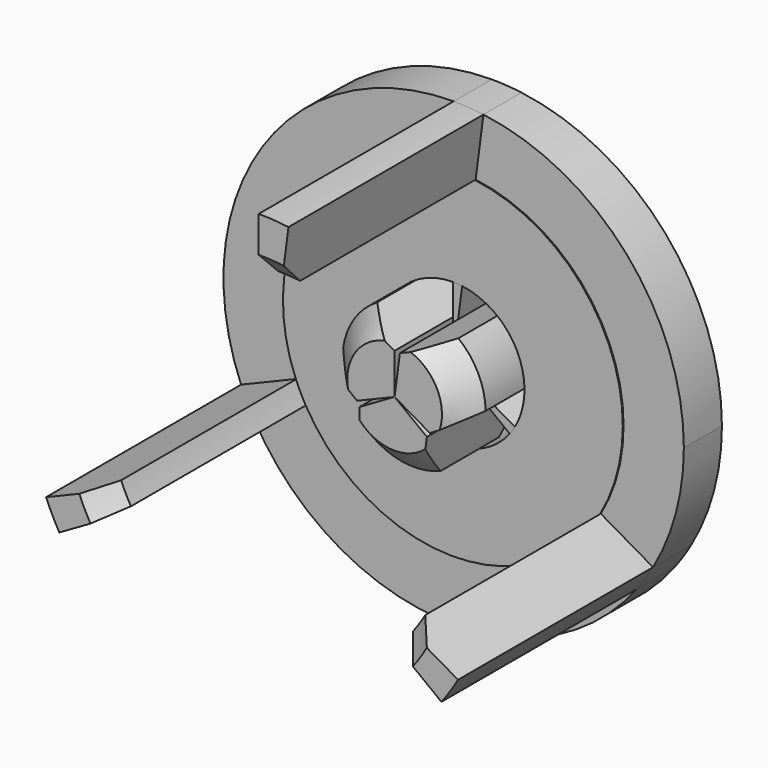
from build123d import *

# Parameters (mm, degrees)
F1_DEPTH      = 60
F2_DEPTH      = 9.8
F3_DEPTH      = 25
F4_DEPTH      = 10
F5_DEPTH      = 10
F6_T1_DEPTH   = 64.9472775058
F6_T4_ANGLE   = 212.5191011757
F6_T6_ANGLE   = 212.5191011757
F6_2_T1_DEPTH = 64.9472775058
F6_2_T4_ANGLE = 212.5191011757
F6_2_T6_ANGLE = 212.5191011757
F6_3_T1_DEPTH = 64.9472775058
F6_3_T4_ANGLE = 212.5191011757
F6_3_T6_ANGLE = 212.5191011757
F7_SIZE       = 5
F7_2_SIZE     = 5
F7_3_SIZE     = 5


# Not quite as in the source:
# - a fillet or chamfer that OpenCascade refuses, or shapes differently, is made with other operations: its cross-section is extruded or revolved along the edge and cut away or added


with BuildPart() as f1:
    # F0 (on Front) → F1 (new body)
    with BuildSketch(Plane.XZ):
        with BuildLine():
            ThreePointArc((0, 35), (2.2707204157, 34.9262627373), (4.5318730195, 34.7053616454))
            Line((4.5318730195, 34.7053616454), (6.1392555161, 47.0147954288))
            ThreePointArc((6.1392555161, 47.0147954288), (3.0761084385, 47.3140465864), (0, 47.4139372706))
            Line((0, 47.4139372706), (0, 35))
        make_face()
    extrude(amount=F1_DEPTH)

    # F7
    f7_edges = [f1.edges().sort_by_distance(p)[0] for p in [
        (2.27072, -60, 34.926263),
    ]]
    chamfer(f7_edges, length=F7_SIZE)


with BuildPart() as f1b:
    # F0 (on Front) → F1, piece 2 (new body)
    with BuildSketch(Plane.XZ):
        with BuildLine():
            Line((41.0616741698, -23.7069686353), (30.3108891325, -17.5))
            ThreePointArc((30.3108891325, -17.5), (29.1116705819, -19.4296329335), (27.7897883227, -21.2773979843))
            Line((27.7897883227, -21.2773979843), (37.646379437, -28.8241489517))
            ThreePointArc((37.646379437, -28.8241489517), (39.4371120804, -26.3210113457), (41.0616741698, -23.7069686353))
        make_face()
    extrude(amount=F1_DEPTH)

    # F7#2
    f7_2_edges = [f1b.edges().sort_by_distance(p)[0] for p in [
        (29.111671, -60, -19.429633),
    ]]
    chamfer(f7_2_edges, length=F7_2_SIZE)


with BuildPart() as f1c:
    # F0 (on Front) → F1, piece 3 (new body)
    with BuildSketch(Plane.XZ):
        with BuildLine():
            ThreePointArc((-30.3108891325, -17.5), (-31.3823909976, -15.4966298038), (-32.3216613422, -13.4279636611))
            Line((-32.3216613422, -13.4279636611), (-43.7856349531, -18.1906464771))
            ThreePointArc((-43.7856349531, -18.1906464771), (-42.5132205189, -20.9930352406), (-41.0616741698, -23.7069686353))
            Line((-41.0616741698, -23.7069686353), (-30.3108891325, -17.5))
        make_face()
    extrude(amount=F1_DEPTH)

    # F7#3
    f7_3_edges = [f1c.edges().sort_by_distance(p)[0] for p in [
        (-31.382391, -60, -15.49663),
    ]]
    chamfer(f7_3_edges, length=F7_3_SIZE)


with BuildPart() as f2:
    # F0 (on Front) → F2 (new body)
    with BuildSketch(Plane.XZ):
        with BuildLine():
            ThreePointArc((4.5318730195, 34.7053616454), (26.3022390271, 23.0909554189), (35, 0))
            ThreePointArc((35, 0), (33.8074039201, -9.0586665786), (30.3108891325, -17.5))
            Line((30.3108891325, -17.5), (41.0616741698, -23.7069686353))
            ThreePointArc((41.0616741698, -23.7069686353), (45.7983465358, -12.2716299689), (47.4139372706, 0))
            ThreePointArc((47.4139372706, 0), (35.6312203232, 31.2809460501), (6.1392555161, 47.0147954288))
            Line((6.1392555161, 47.0147954288), (4.5318730195, 34.7053616454))
        make_face()
        with BuildLine():
            ThreePointArc((0, 35), (2.2707204157, 34.9262627373), (4.5318730195, 34.7053616454))
            Line((4.5318730195, 34.7053616454), (6.1392555161, 47.0147954288))
            ThreePointArc((6.1392555161, 47.0147954288), (3.0761084385, 47.3140465864), (0, 47.4139372706))
            Line((0, 47.4139372706), (0, 35))
        make_face()
        with BuildLine():
            Line((41.0616741698, -23.7069686353), (30.3108891325, -17.5))
            ThreePointArc((30.3108891325, -17.5), (29.1116705819, -19.4296329335), (27.7897883227, -21.2773979843))
            Line((27.7897883227, -21.2773979843), (37.646379437, -28.8241489517))
            ThreePointArc((37.646379437, -28.8241489517), (39.4371120804, -26.3210113457), (41.0616741698, -23.7069686353))
        make_face()
        with BuildLine():
            ThreePointArc((-32.3216613422, -13.4279636611), (-29.1116705819, 19.4296329335), (0, 35))
            Line((0, 35), (0, 47.4139372706))
            ThreePointArc((0, 47.4139372706), (-39.4371120804, 26.3210113457), (-43.7856349531, -18.1906464771))
            Line((-43.7856349531, -18.1906464771), (-32.3216613422, -13.4279636611))
        make_face()
        with BuildLine():
            Line((37.646379437, -28.8241489517), (27.7897883227, -21.2773979843))
            ThreePointArc((27.7897883227, -21.2773979843), (-2.2707204157, -34.9262627373), (-30.3108891325, -17.5))
            Line((-30.3108891325, -17.5), (-41.0616741698, -23.7069686353))
            ThreePointArc((-41.0616741698, -23.7069686353), (-3.0761084385, -47.3140465864), (37.646379437, -28.8241489517))
        make_face()
        with BuildLine():
            ThreePointArc((-30.3108891325, -17.5), (-31.3823909976, -15.4966298038), (-32.3216613422, -13.4279636611))
            Line((-32.3216613422, -13.4279636611), (-43.7856349531, -18.1906464771))
            ThreePointArc((-43.7856349531, -18.1906464771), (-42.5132205189, -20.9930352406), (-41.0616741698, -23.7069686353))
            Line((-41.0616741698, -23.7069686353), (-30.3108891325, -17.5))
        make_face()
    extrude(amount=F2_DEPTH)


with BuildPart() as f3:
    # F0 (on Front) → F3 (new body)
    with BuildSketch(Plane.XZ):
        with BuildLine():
            Line((0, 0), (0, 14.75))
            ThreePointArc((0, 14.75), (-12.2684897452, 8.1882024506), (-13.6212715656, -5.6589275429))
            Line((-13.6212715656, -5.6589275429), (0, 0))
        make_face()
    extrude(amount=F3_DEPTH)

    # F6: chamfer of 5 on 4 edges, made by hand

    # F6_s2 → F6_t1 (cut)
    with BuildSketch(Plane.XZ.offset(-19.9736387529)):
        with BuildLine():
            Line((0, 8.3703345214), (-7.5641025641, 12.6628137631))
            ThreePointArc((-7.5641025641, 12.6628137631), (-3.9937030678, 14.1990434821), (0, 14.75))
            Line((0, 14.75), (0, 8.3703345214))
        make_face()
        with BuildLine():
            Line((-7.7298033635, -3.2113299367), (-14.5958192129, 2.1271016679))
            ThreePointArc((-14.5958192129, 2.1271016679), (-14.6446849851, -1.759460624), (-13.6212715656, -5.6589275429))
            Line((-13.6212715656, -5.6589275429), (-7.7298033635, -3.2113299367))
        make_face()
    extrude(amount=F6_T1_DEPTH, mode=Mode.SUBTRACT)

    # F6_s3 → F6_t4 (revolve, cut)
    with BuildSketch(Plane(origin=(0, 0, 0), x_dir=(0, 1, 0), z_dir=(0.6430632155, 0, -0.7658130979))):
        Polygon((-5, 14.75), (0, 9.75), (0, 14.75), align=None)
    revolve(axis=Axis((0, 0, 0), (0, -1, 0)), revolution_arc=F6_T4_ANGLE, mode=Mode.SUBTRACT)

    # F6_s5 → F6_t6 (revolve, cut)
    with BuildSketch(Plane(origin=(0, 0, 0), x_dir=(0, 1, 0), z_dir=(0.6430632155, 0, -0.7658130979))):
        Polygon((-20, 14.75), (-25, 9.75), (-25, 14.75), align=None)
    revolve(axis=Axis((0, -25, 0), (0, -1, 0)), revolution_arc=F6_T6_ANGLE, mode=Mode.SUBTRACT)


with BuildPart() as f3b:
    # F0 (on Front) → F3, piece 2 (new body)
    with BuildSketch(Plane.XZ):
        with BuildLine():
            ThreePointArc((14.75, 0), (11.0845150186, 9.7311883551), (1.9098607725, 14.6258309791))
            Line((1.9098607725, 14.6258309791), (0, 0))
            Line((0, 0), (12.7738747058, -7.375))
            ThreePointArc((12.7738747058, -7.375), (14.2474059378, -3.8175809153), (14.75, 0))
        make_face()
    extrude(amount=F3_DEPTH)

    # F6#2: chamfer of 5 on 4 edges, made by hand

    # F6_2_s2 → F6_2_t1 (cut)
    with BuildSketch(Plane.XZ.offset(-19.9736387529)):
        with BuildLine():
            Line((7.2489223337, -4.1851672607), (14.7483696843, 0.2192980958))
            ThreePointArc((14.7483696843, 0.2192980958), (14.2935838988, -3.6408734291), (12.7738747058, -7.375))
            Line((12.7738747058, -7.375), (7.2489223337, -4.1851672607))
        make_face()
        with BuildLine():
            Line((1.0838083766, 8.2998710474), (9.1400336873, 11.5767993934))
            ThreePointArc((9.1400336873, 11.5767993934), (5.7986048952, 13.5623995395), (1.9098607725, 14.6258309791))
            Line((1.9098607725, 14.6258309791), (1.0838083766, 8.2998710474))
        make_face()
    extrude(amount=F6_2_T1_DEPTH, mode=Mode.SUBTRACT)

    # F6_2_s3 → F6_2_t4 (revolve, cut)
    with BuildSketch(Plane(origin=(0, 0, 0), x_dir=(0, 1, 0), z_dir=(-0.7368088334, 0, -0.6761011337))):
        Polygon((-25, -9.75), (-20, -14.75), (-25, -14.75), align=None)
    revolve(axis=Axis((0, -25, 0), (0, 1, 0)), revolution_arc=F6_2_T4_ANGLE, mode=Mode.SUBTRACT)

    # F6_2_s5 → F6_2_t6 (revolve, cut)
    with BuildSketch(Plane(origin=(0, 0, 0), x_dir=(0, 1, 0), z_dir=(-0.9847452051, 0, -0.1740025319))):
        Polygon((0, 9.75), (-5, 14.75), (0, 14.75), align=None)
    revolve(axis=Axis((0, 0, 0), (0, -1, 0)), revolution_arc=F6_2_T6_ANGLE, mode=Mode.SUBTRACT)


with BuildPart() as f3c:
    # F0 (on Front) → F3, piece 3 (new body)
    with BuildSketch(Plane.XZ):
        with BuildLine():
            Line((11.7114107931, -8.9669034362), (0, 0))
            Line((0, 0), (-12.7738747058, -7.375))
            ThreePointArc((-12.7738747058, -7.375), (-0.9569464609, -14.7189250107), (11.7114107931, -8.9669034362))
        make_face()
    extrude(amount=F3_DEPTH)

    # F6#3: chamfer of 5 on 4 edges, made by hand

    # F6_3_s2 → F6_3_t1 (cut)
    with BuildSketch(Plane.XZ.offset(-19.9736387529)):
        with BuildLine():
            Line((-7.2489223337, -4.1851672607), (-7.1842671202, -12.8821118589))
            ThreePointArc((-7.1842671202, -12.8821118589), (-10.299880831, -10.558170053), (-12.7738747058, -7.375))
            Line((-12.7738747058, -7.375), (-7.2489223337, -4.1851672607))
        make_face()
        with BuildLine():
            Line((6.6459949868, -5.0885411107), (5.4557855256, -13.7039010613))
            ThreePointArc((5.4557855256, -13.7039010613), (8.8460800899, -11.8029389155), (11.7114107931, -8.9669034362))
            Line((11.7114107931, -8.9669034362), (6.6459949868, -5.0885411107))
        make_face()
    extrude(amount=F6_3_T1_DEPTH, mode=Mode.SUBTRACT)

    # F6_3_s3 → F6_3_t4 (revolve, cut)
    with BuildSketch(Plane(origin=(0, 0, 0), x_dir=(0, 1, 0), z_dir=(0.3416819896, 0, 0.9398156298))):
        Polygon((-20, 14.75), (-25, 9.75), (-25, 14.75), align=None)
    revolve(axis=Axis((0, -25, 0), (0, -1, 0)), revolution_arc=F6_3_T4_ANGLE, mode=Mode.SUBTRACT)

    # F6_3_s5 → F6_3_t6 (revolve, cut)
    with BuildSketch(Plane(origin=(0, 0, 0), x_dir=(0, 1, 0), z_dir=(0.3416819896, 0, 0.9398156298))):
        Polygon((-5, 14.75), (0, 9.75), (0, 14.75), align=None)
    revolve(axis=Axis((0, 0, 0), (0, -1, 0)), revolution_arc=F6_3_T6_ANGLE, mode=Mode.SUBTRACT)


with BuildPart() as f4:
    # F0 (on Front) → F4 (new body)
    with BuildSketch(Plane.XZ):
        with BuildLine():
            ThreePointArc((-30.3108891325, -17.5), (-2.2707204157, -34.9262627373), (27.7897883227, -21.2773979843))
            Line((27.7897883227, -21.2773979843), (11.7114107931, -8.9669034362))
            ThreePointArc((11.7114107931, -8.9669034362), (-0.9569464609, -14.7189250107), (-12.7738747058, -7.375))
            Line((-12.7738747058, -7.375), (-30.3108891325, -17.5))
        make_face()
        with BuildLine():
            ThreePointArc((30.3108891325, -17.5), (33.8074039201, -9.0586665786), (35, 0))
            ThreePointArc((35, 0), (26.3022390271, 23.0909554189), (4.5318730195, 34.7053616454))
            Line((4.5318730195, 34.7053616454), (1.9098607725, 14.6258309791))
            ThreePointArc((1.9098607725, 14.6258309791), (11.0845150186, 9.7311883551), (14.75, 0))
            ThreePointArc((14.75, 0), (14.2474059378, -3.8175809153), (12.7738747058, -7.375))
            Line((12.7738747058, -7.375), (30.3108891325, -17.5))
        make_face()
        with BuildLine():
            ThreePointArc((27.7897883227, -21.2773979843), (29.1116705819, -19.4296329335), (30.3108891325, -17.5))
            Line((30.3108891325, -17.5), (12.7738747058, -7.375))
            ThreePointArc((12.7738747058, -7.375), (12.2684897452, -8.1882024506), (11.7114107931, -8.9669034362))
            Line((11.7114107931, -8.9669034362), (27.7897883227, -21.2773979843))
        make_face()
        with BuildLine():
            Line((-13.6212715656, -5.6589275429), (-32.3216613422, -13.4279636611))
            ThreePointArc((-32.3216613422, -13.4279636611), (-31.3823909976, -15.4966298038), (-30.3108891325, -17.5))
            Line((-30.3108891325, -17.5), (-12.7738747058, -7.375))
            ThreePointArc((-12.7738747058, -7.375), (-13.2254362061, -6.5307225602), (-13.6212715656, -5.6589275429))
        make_face()
        with BuildLine():
            Line((0, 14.75), (0, 35))
            ThreePointArc((0, 35), (-29.1116705819, 19.4296329335), (-32.3216613422, -13.4279636611))
            Line((-32.3216613422, -13.4279636611), (-13.6212715656, -5.6589275429))
            ThreePointArc((-13.6212715656, -5.6589275429), (-12.2684897452, 8.1882024506), (0, 14.75))
        make_face()
        with BuildLine():
            Line((1.9098607725, 14.6258309791), (4.5318730195, 34.7053616454))
            ThreePointArc((4.5318730195, 34.7053616454), (2.2707204157, 34.9262627373), (0, 35))
            Line((0, 35), (0, 14.75))
            ThreePointArc((0, 14.75), (0.9569464609, 14.7189250107), (1.9098607725, 14.6258309791))
        make_face()
    extrude(amount=F4_DEPTH)


with BuildPart() as f5:
    # F0 (on Front) → F5 (new body)
    with BuildSketch(Plane.XZ):
        with BuildLine():
            ThreePointArc((11.7114107931, -8.9669034362), (12.2684897452, -8.1882024506), (12.7738747058, -7.375))
            Line((12.7738747058, -7.375), (0, 0))
            Line((0, 0), (11.7114107931, -8.9669034362))
        make_face()
    extrude(amount=F5_DEPTH)


with BuildPart() as f5b:
    # F0 (on Front) → F5, piece 2 (new body)
    with BuildSketch(Plane.XZ):
        with BuildLine():
            Line((-12.7738747058, -7.375), (0, 0))
            Line((0, 0), (-13.6212715656, -5.6589275429))
            ThreePointArc((-13.6212715656, -5.6589275429), (-13.2254362061, -6.5307225602), (-12.7738747058, -7.375))
        make_face()
    extrude(amount=F5_DEPTH)


with BuildPart() as f5c:
    # F0 (on Front) → F5, piece 3 (new body)
    with BuildSketch(Plane.XZ):
        with BuildLine():
            Line((0, 0), (1.9098607725, 14.6258309791))
            ThreePointArc((1.9098607725, 14.6258309791), (0.9569464609, 14.7189250107), (0, 14.75))
            Line((0, 14.75), (0, 0))
        make_face()
    extrude(amount=F5_DEPTH)


solid = Compound([f1.part, f1b.part, f1c.part, f2.part, f3.part, f3b.part, f3c.part, f4.part, f5.part, f5b.part, f5c.part])
